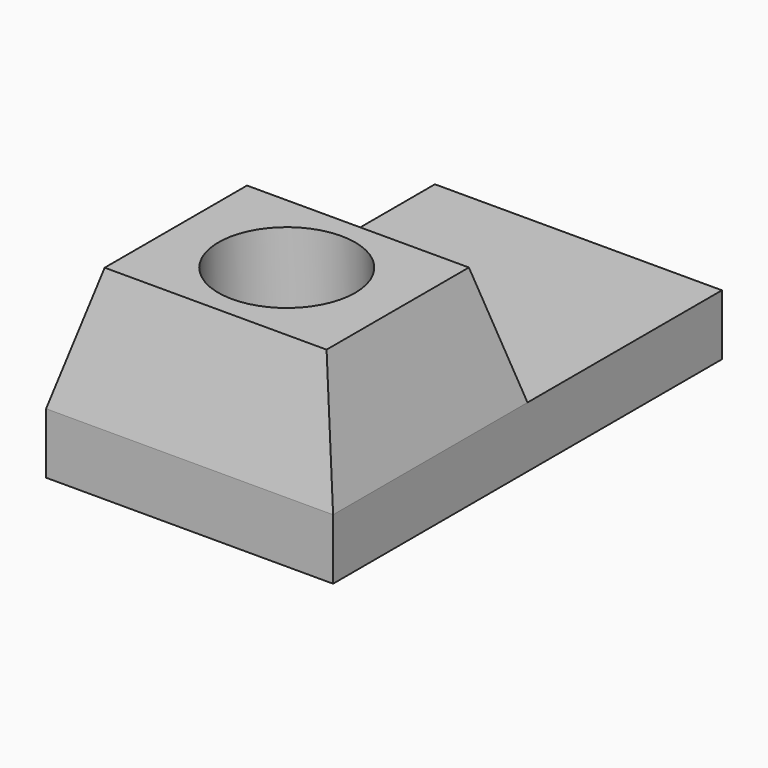
from build123d import *

# Parameters (mm, degrees)
F0_W     = 59.9948
F0_H     = 12.7
F1_DEPTH = 101.6
F2_W     = 59.9948
F2_H     = 50.8
F3_DEPTH = 25.4
F3_TAPER = 15
F4_R     = 14.2909740927
F5_DEPTH = 19.05


with BuildPart() as f1:
    # F0 (on Front) → F1 (new body)
    with BuildSketch(Plane.XZ):
        with Locations((2.9941368848, -8.3058523926)):
            Rectangle(F0_W, F0_H)
    extrude(amount=F1_DEPTH)

    # F2 (on face) → F3 (join)
    with BuildSketch(Plane.XY.offset(-1.9558523926)):
        with Locations((2.9941368848, -76.2)):
            Rectangle(F2_W, F2_H)
    extrude(amount=F3_DEPTH, taper=F3_TAPER)

    # F4 (on face) → F5 (cut)
    with BuildSketch(Plane.XY.offset(23.4441476074)):
        with Locations((2.9941368848, -76.2)):
            Circle(F4_R)
    extrude(amount=-F5_DEPTH, mode=Mode.SUBTRACT)


solid = f1.part
